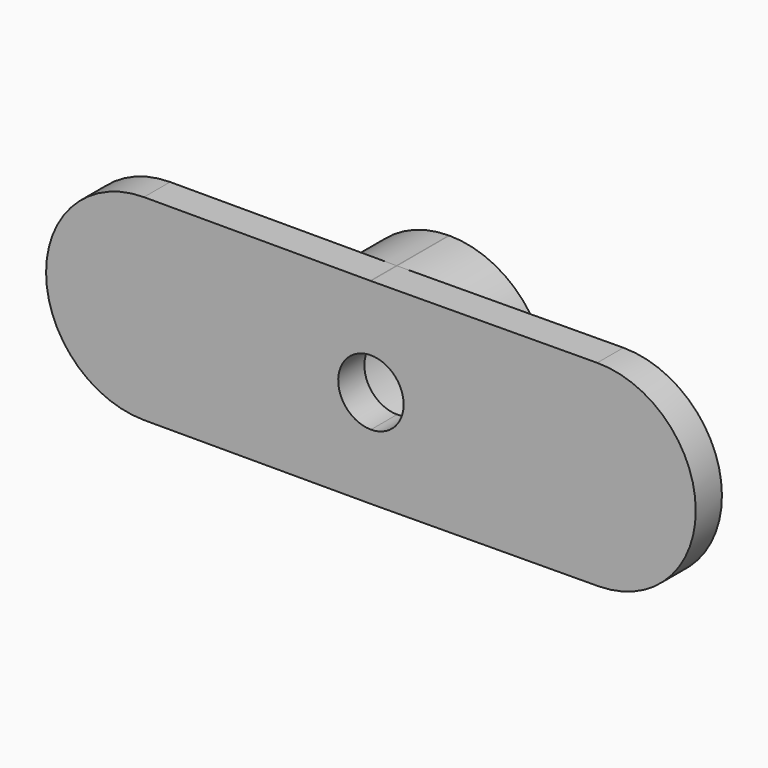
from build123d import *
from build123d import SkipClean  # not in build123d's __all__

# Parameters (mm, degrees)
F1_DEPTH = 19.05
F2_DEPTH = 12.7
F3_DEPTH = 12.7


with BuildPart() as f1:
    # F0 (on Front) → F1 (new body)
    with BuildSketch(Plane.XZ):
        with BuildLine():
            ThreePointArc((61.5727165116, -19.0499999988), (61.5728220467, -19.0499999997), (61.5729275818, -19.05))
            ThreePointArc((61.5729275818, -19.05), (61.6368837688, -19.0498926403), (61.7008392349, -19.0495705623))
            ThreePointArc((61.7008392349, -19.0495705623), (80.6228005597, 0.0695667009), (61.5617064856, 19.0499966952))
            ThreePointArc((61.5617064856, 19.0499966952), (61.5090769294, 19.0498929943), (61.4564478606, 19.0496438936))
            ThreePointArc((61.4564478606, 19.0496438936), (42.4051790983, 0.0593448366), (61.3370395323, -19.0499973876))
            Line((61.3370395323, -19.0499973876), (61.5727165116, -19.0499999988))
        make_face()
        with BuildLine():
            ThreePointArc((61.5729275818, -12.7), (52.5926714608, 8.9802561211), (74.2729275818, 0))
            ThreePointArc((74.2729275818, 0), (70.5531837029, -8.9802561211), (61.5729275818, -12.7))
        make_face(mode=Mode.SUBTRACT)
        with BuildLine():
            ThreePointArc((61.3370395323, -19.0499973876), (61.4548780179, -19.0503631562), (61.5727165116, -19.0499999988))
            Line((61.5727165116, -19.0499999988), (61.3370395323, -19.0499973876))
        make_face()
        with BuildLine():
            ThreePointArc((61.5617064856, 19.0499966952), (80.6228005597, 0.0695667009), (61.7008392349, -19.0495705623))
            Line((61.7008392349, -19.0495705623), (105.7561740171, -18.7537533585))
            ThreePointArc((105.7561740171, -18.7537533585), (124.6268697008, 0.4243875569), (105.5006242064, 19.3476794968))
            Line((105.5006242064, 19.3476794968), (61.5617064856, 19.0499966952))
        make_face()
        with BuildLine():
            Line((17.5163885853, -19.0495118633), (61.3370395323, -19.0499973876))
            ThreePointArc((61.3370395323, -19.0499973876), (42.4051790983, 0.0593448366), (61.4564478606, 19.0496438936))
            Line((61.4564478606, 19.0496438936), (17.516521874, 19.0527779802))
            ThreePointArc((17.516521874, 19.0527779802), (-1.4824426783, 0.0016995201), (17.5163885853, -19.0495118633))
        make_face()
        with BuildLine():
            ThreePointArc((61.5729275818, -12.7), (70.5531837029, -8.9802561211), (74.2729275818, 0))
            ThreePointArc((74.2729275818, 0), (52.5926714608, 8.9802561211), (61.5729275818, -12.7))
        make_face()
        with BuildLine():
            ThreePointArc((67.9229275818, 0), (66.0630556424, -4.4901280605), (61.5729275818, -6.35))
            ThreePointArc((61.5729275818, -6.35), (57.0827995213, 4.4901280605), (67.9229275818, 0))
        make_face(mode=Mode.SUBTRACT)
    extrude(amount=F1_DEPTH)

    # F0 (on Front) → F2 (cut)
    with BuildSketch(Plane.XZ):
        with BuildLine():
            ThreePointArc((61.5729275818, -12.7), (70.5531837029, -8.9802561211), (74.2729275818, 0))
            ThreePointArc((74.2729275818, 0), (52.5926714608, 8.9802561211), (61.5729275818, -12.7))
        make_face()
        with BuildLine():
            ThreePointArc((67.9229275818, 0), (66.0630556424, -4.4901280605), (61.5729275818, -6.35))
            ThreePointArc((61.5729275818, -6.35), (57.0827995213, 4.4901280605), (67.9229275818, 0))
        make_face(mode=Mode.SUBTRACT)
        with BuildLine():
            Line((17.5163885853, -19.0495118633), (61.3370395323, -19.0499973876))
            ThreePointArc((61.3370395323, -19.0499973876), (42.4051790983, 0.0593448366), (61.4564478606, 19.0496438936))
            Line((61.4564478606, 19.0496438936), (17.516521874, 19.0527779802))
            ThreePointArc((17.516521874, 19.0527779802), (-1.4824426783, 0.0016995201), (17.5163885853, -19.0495118633))
        make_face()
    extrude(amount=F2_DEPTH, mode=Mode.SUBTRACT)

    # F0 (on Front) → F3 (cut)
    with BuildSketch(Plane.XZ):
        with BuildLine():
            ThreePointArc((61.5617064856, 19.0499966952), (80.6228005597, 0.0695667009), (61.7008392349, -19.0495705623))
            Line((61.7008392349, -19.0495705623), (105.7561740171, -18.7537533585))
            ThreePointArc((105.7561740171, -18.7537533585), (124.6268697008, 0.4243875569), (105.5006242064, 19.3476794968))
            Line((105.5006242064, 19.3476794968), (61.5617064856, 19.0499966952))
        make_face()
    with SkipClean():  # cleaning this boolean's faces spoils the solid; the shape is the same uncleaned
        extrude(amount=F3_DEPTH, mode=Mode.SUBTRACT)


solid = f1.part
